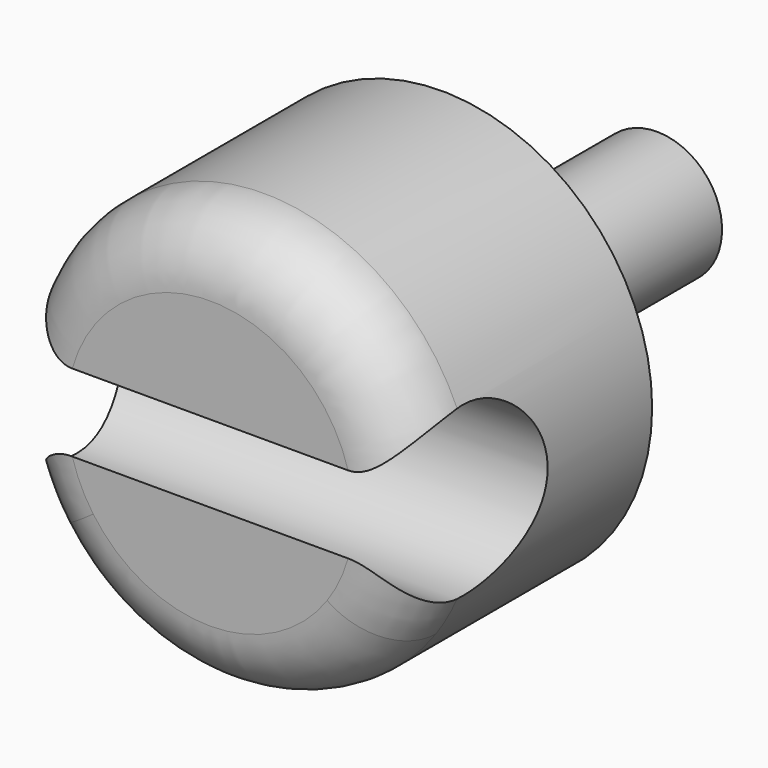
from build123d import *

# Parameters (mm, degrees)
F0_R        = 31.2849976613
F1_DEPTH    = 43
F2_R        = 12.5
F3_DEPTH    = 40
F4_T3_ANGLE = 250.4726360275
F4_T6_ANGLE = 250.4726360275
F5_R        = 9.6724066991
F6_DEPTH    = 40


# Not quite as in the source:
# - a fillet or chamfer that OpenCascade refuses, or shapes differently, is made with other operations: its cross-section is extruded or revolved along the edge and cut away or added


with BuildPart() as f1:
    # F0 (on Front) → F1 (new body)
    with BuildSketch(Plane.XZ):
        with Locations((3.0078960117, 0)):
            Circle(F0_R)
    extrude(amount=F1_DEPTH)

    # F2 (on Right) → F3 (cut, symmetric)
    with BuildSketch(Plane.YZ):
        with Locations((-31.9053208832, 0)):
            Circle(F2_R)
    extrude(amount=F3_DEPTH, both=True, mode=Mode.SUBTRACT)

    # F4: fillet of radius 10 on 2 edges, made by hand


with BuildPart() as f4_tool1:
    # F4_s2 → F4_t3 (revolve)
    with BuildSketch(Plane(origin=(1.0012428292, 0, 1.4174438647), x_dir=(0, 1, 0), z_dir=(-0.5769501631, 0, -0.8167793517))):
        with BuildLine():
            ThreePointArc((-33, 33.7417850156), (-40.0710678119, 30.8128528275), (-43, 23.7417850156))
            Line((-43, 23.7417850156), (-43, 33.7417850156))
            Line((-43, 33.7417850156), (-33, 33.7417850156))
        make_face()
    revolve(axis=Axis((3.0078960117, -43, 0), (0, -1, 0)), revolution_arc=F4_T3_ANGLE)


with BuildPart() as f4_tool4:
    # F4_s5 → F4_t6 (revolve)
    with BuildSketch(Plane(origin=(1.0012428292, 0, 1.4174438647), x_dir=(0, 1, 0), z_dir=(0.5769501631, 0, 0.8167793517))):
        with BuildLine():
            ThreePointArc((-33, 28.828210307), (-40.0710678119, 25.8992781188), (-43, 18.828210307))
            Line((-43, 18.828210307), (-43, 28.828210307))
            Line((-43, 28.828210307), (-33, 28.828210307))
        make_face()
    revolve(axis=Axis((3.0078960117, -43, 0), (0, -1, 0)), revolution_arc=F4_T6_ANGLE)


with BuildPart() as f1_1:
    add(f1.part)

    # F4_t7: cut F4_tool1, F4_tool4
    add([f4_tool1.part, f4_tool4.part], mode=Mode.SUBTRACT)

    # F5 (on face) → F6 (join)
    with BuildSketch(Plane(origin=(0, 0, 0), x_dir=(-1, 0, 0), z_dir=(0, 1, 0))):
        with Locations((-3.0078960117, 0)):
            Circle(F5_R)
    extrude(amount=F6_DEPTH)


solid = f1_1.part
